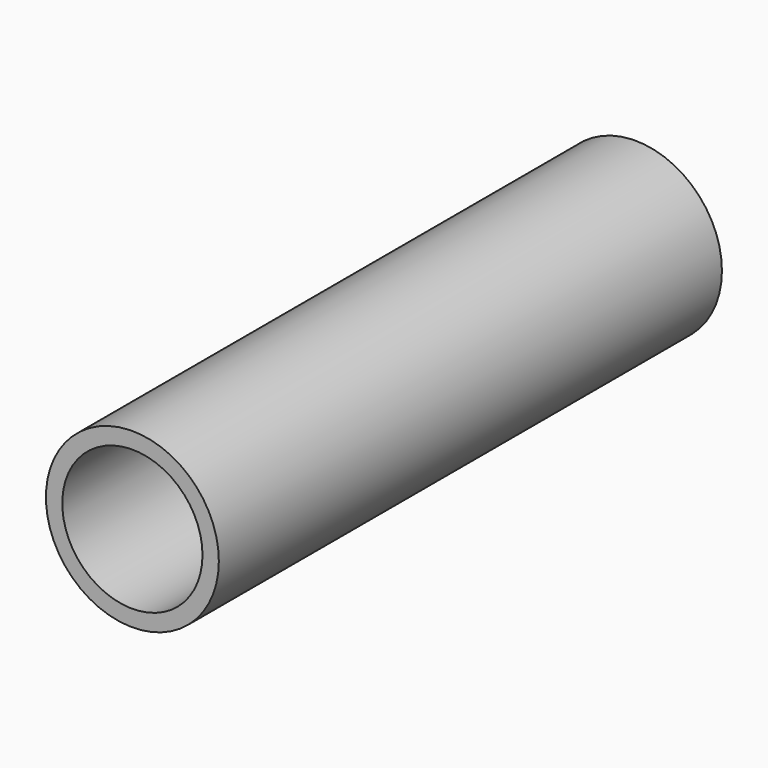
from build123d import *

# Parameters (mm, degrees)
F0_R     = 27.5
F0_R_2   = 22.3002892969
F1_DEPTH = 100


with BuildPart() as f1:
    # F0 (on Front) → F1 (new body, symmetric)
    with BuildSketch(Plane.XZ):
        Circle(F0_R)
        Circle(F0_R_2, mode=Mode.SUBTRACT)
    extrude(amount=F1_DEPTH, both=True)


solid = f1.part
